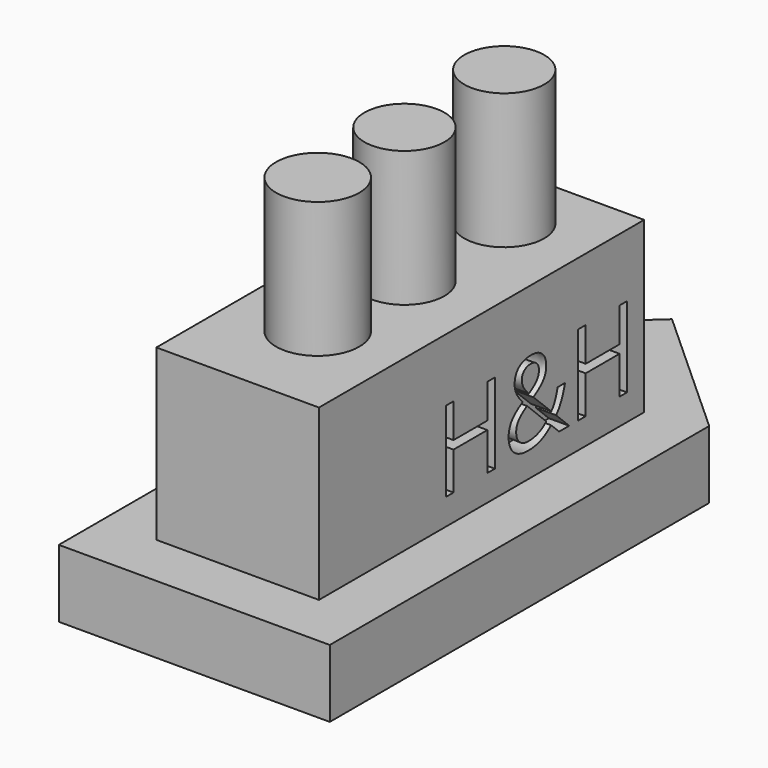
from build123d import *

# Parameters (mm, degrees)
F1_DEPTH     = 10
F2_W         = 24
F2_H         = 60
F3_DEPTH     = 25
F5_R         = 5.9030434055
F5_R_2       = 6.1444875752
F5_R_3       = 5.9030426011
F6_DEPTH     = 20
F8_TEXT_SIZE = 16.6142799167
F9_DEPTH     = 3


# Not quite as in the source:
# - Text() gives the source's letters only with a copy of the font that has no kerning and outlines rounded to 1/6400 em; it was checked with that copy


with BuildPart() as f1:
    # F0 (on Top) → F1 (new body)
    with BuildSketch(Plane.XY):
        Polygon((0, 65.3696756456), (-20, 47.2313184984), (-20, -22.7686815016), (20, -22.7686815016), (20, 47.2313184984), align=None)
    extrude(amount=F1_DEPTH)

    # F2 (on face) → F3 (join)
    with BuildSketch(Plane.XY.offset(10)):
        with Locations((0, 15.2313184984)):
            Rectangle(F2_W, F2_H)
    extrude(amount=F3_DEPTH)

    # F5 (on face) → F6 (join)
    with BuildSketch(Plane.XY.offset(35)):
        with Locations((0, 34.4177186489)):
            Circle(F5_R)
        Circle(F5_R_2)
        with Locations((0, 16.0049479455)):
            Circle(F5_R_3)
    extrude(amount=F6_DEPTH)

    # F8 (on face) → F9 (cut)
    with BuildSketch(Plane.YZ.offset(12)):
        with Locations((7.0504047908, 13.8594247401)):
            Text('H&H', F8_TEXT_SIZE, font='Open Sans', text_align=(TextAlign.LEFT, TextAlign.BOTTOM))
    extrude(amount=-F9_DEPTH, mode=Mode.SUBTRACT)


solid = f1.part
